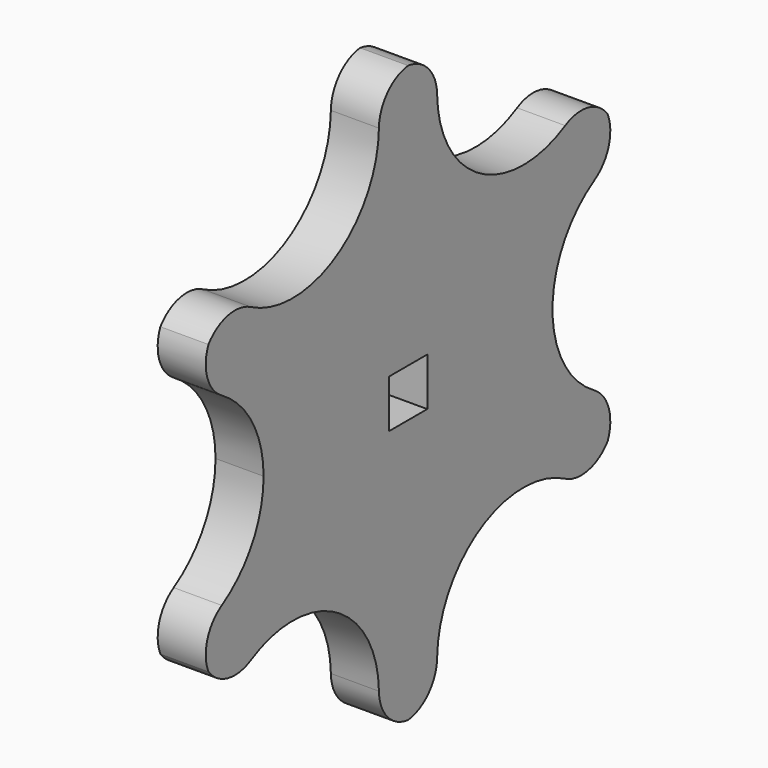
from build123d import *

# Parameters (mm, degrees)
F1_DEPTH    = 3.175
F2_W        = 3.175
F2_H        = 3.175
F3_DEPTH    = 25.4
F4_T1_DEPTH = 19.0841031127


# Not quite as in the source:
# - a fillet or chamfer that OpenCascade refuses, or shapes differently, is made with other operations: its cross-section is extruded or revolved along the edge and cut away or added


with BuildPart() as f1:
    # F0 (on Right) → F1 (new body)
    with BuildSketch(Plane.YZ):
        with BuildLine():
            ThreePointArc((17.7183197491, -6.9974027515), (11.9270078227, 0), (17.7183197491, 6.9974027515))
            ThreePointArc((17.7183197491, 6.9974027515), (16.4977839421, 9.525), (14.9190884179, 11.8458136394))
            ThreePointArc((14.9190884179, 11.8458136394), (5.9635039114, 10.3290917656), (2.7992313312, 18.8432163909))
            ThreePointArc((2.7992313312, 18.8432163909), (0, 19.05), (-2.7992313312, 18.8432163909))
            ThreePointArc((-2.7992313312, 18.8432163909), (-2.5020157635, 17.6871997533), (-2.4020078227, 16.4977839421))
            ThreePointArc((-2.4020078227, 16.4977839421), (-7.0435721899, 9.8209932773), (-14.9190884179, 11.8458136394))
            ThreePointArc((-14.9190884179, 11.8458136394), (-16.4977839421, 9.525), (-17.7183197491, 6.9974027515))
            ThreePointArc((-17.7183197491, 6.9974027515), (-13.5626251464, 4.5415564264), (-11.9270078227, 0))
            ThreePointArc((-11.9270078227, 0), (-13.5626251464, -4.5415564264), (-17.7183197491, -6.9974027515))
            ThreePointArc((-17.7183197491, -6.9974027515), (-16.4977839421, -9.525), (-14.9190884179, -11.8458136394))
            ThreePointArc((-14.9190884179, -11.8458136394), (-7.0435721899, -9.8209932773), (-2.4020078227, -16.4977839421))
            ThreePointArc((-2.4020078227, -16.4977839421), (-2.5020157635, -17.6871997533), (-2.7992313312, -18.8432163909))
            ThreePointArc((-2.7992313312, -18.8432163909), (0, -19.05), (2.7992313312, -18.8432163909))
            ThreePointArc((2.7992313312, -18.8432163909), (5.9635039114, -10.3290917656), (14.9190884179, -11.8458136394))
            ThreePointArc((14.9190884179, -11.8458136394), (16.4977839421, -9.525), (17.7183197491, -6.9974027515))
        make_face()
    extrude(amount=F1_DEPTH)

    # F2 (on face) → F3 (cut)
    with BuildSketch(Plane(origin=(0, 0, 0), x_dir=(0, -1, 0), z_dir=(-1, 0, 0))):
        Rectangle(F2_W, F2_H)
    extrude(amount=-F3_DEPTH, mode=Mode.SUBTRACT)

    # F4: fillet of radius 2.7258813335 on 12 edges, made by hand

    # F4_s2 → F4_t1 (cut)
    with BuildSketch(Plane.YZ.offset(-7.9545515563)):
        with BuildLine():
            ThreePointArc((-16.6826195947, 9.1974291766), (-15.0505041811, 10.5005937812), (-12.9751564545, 10.2661358457))
            ThreePointArc((-12.9751564545, 10.2661358457), (-14.0171055557, 10.9698543809), (-14.9190884179, 11.8458136394))
            ThreePointArc((-14.9190884179, 11.8458136394), (-15.8562439561, 10.5585049892), (-16.6826195947, 9.1974291766))
        make_face()
        with BuildLine():
            ThreePointArc((-15.3783126684, 6.1037471848), (-16.6190330599, 7.78382207), (-16.3065171138, 9.8488577824))
            ThreePointArc((-16.3065171138, 9.8488577824), (-17.0720555246, 8.45265758), (-17.7183197491, 6.9974027515))
            ThreePointArc((-17.7183197491, 6.9974027515), (-16.5087253475, 6.6542423084), (-15.3783126684, 6.1037471848))
        make_face()
        with BuildLine():
            ThreePointArc((-16.3065171138, -9.8488577824), (-16.6190330599, -7.78382207), (-15.3783126684, -6.1037471848))
            ThreePointArc((-15.3783126684, -6.1037471848), (-16.5087253475, -6.6542423084), (-17.7183197491, -6.9974027515))
            ThreePointArc((-17.7183197491, -6.9974027515), (-17.0720555246, -8.45265758), (-16.3065171138, -9.8488577824))
        make_face()
        with BuildLine():
            ThreePointArc((-12.9751564545, -10.2661358457), (-15.0505041811, -10.5005937812), (-16.6826195947, -9.1974291766))
            ThreePointArc((-16.6826195947, -9.1974291766), (-15.8562439561, -10.5585049892), (-14.9190884179, -11.8458136394))
            ThreePointArc((-14.9190884179, -11.8458136394), (-14.0171055557, -10.9698543809), (-12.9751564545, -10.2661358457))
        make_face()
        with BuildLine():
            ThreePointArc((-2.4031562138, -16.3698830306), (-1.5685288788, -18.2844158512), (0.3761024809, -19.046286959))
            ThreePointArc((0.3761024809, -19.046286959), (-1.2158115686, -19.0111625691), (-2.7992313312, -18.8432163909))
            ThreePointArc((-2.7992313312, -18.8432163909), (-2.4916197918, -17.6240966892), (-2.4031562138, -16.3698830306))
        make_face()
        with BuildLine():
            ThreePointArc((-2.4031562138, 16.3698830306), (-1.5685288788, 18.2844158512), (0.3761024809, 19.046286959))
            ThreePointArc((0.3761024809, 19.046286959), (-1.2158115686, 19.0111625691), (-2.7992313312, 18.8432163909))
            ThreePointArc((-2.7992313312, 18.8432163909), (-2.4916197918, 17.6240966892), (-2.4031562138, 16.3698830306))
        make_face()
        with BuildLine():
            ThreePointArc((16.6826195947, 9.1974291766), (15.0505041811, 10.5005937812), (12.9751564545, 10.2661358457))
            ThreePointArc((12.9751564545, 10.2661358457), (14.0171055557, 10.9698543809), (14.9190884179, 11.8458136394))
            ThreePointArc((14.9190884179, 11.8458136394), (15.8562439561, 10.5585049892), (16.6826195947, 9.1974291766))
        make_face()
        with BuildLine():
            ThreePointArc((-0.3761024809, 19.046286959), (1.5685288788, 18.2844158512), (2.4031562138, 16.3698830306))
            ThreePointArc((2.4031562138, 16.3698830306), (2.4916197918, 17.6240966892), (2.7992313312, 18.8432163909))
            ThreePointArc((2.7992313312, 18.8432163909), (1.2158115686, 19.0111625691), (-0.3761024809, 19.046286959))
        make_face()
        with BuildLine():
            ThreePointArc((15.3783126684, 6.1037471848), (16.6190330599, 7.78382207), (16.3065171138, 9.8488577824))
            ThreePointArc((16.3065171138, 9.8488577824), (17.0720555246, 8.45265758), (17.7183197491, 6.9974027515))
            ThreePointArc((17.7183197491, 6.9974027515), (16.5087253475, 6.6542423084), (15.3783126684, 6.1037471848))
        make_face()
        with BuildLine():
            ThreePointArc((16.3065171138, -9.8488577824), (16.6190330599, -7.78382207), (15.3783126684, -6.1037471848))
            ThreePointArc((15.3783126684, -6.1037471848), (16.5087253475, -6.6542423084), (17.7183197491, -6.9974027515))
            ThreePointArc((17.7183197491, -6.9974027515), (17.0720555246, -8.45265758), (16.3065171138, -9.8488577824))
        make_face()
        with BuildLine():
            ThreePointArc((12.9751564545, -10.2661358457), (15.0505041811, -10.5005937812), (16.6826195947, -9.1974291766))
            ThreePointArc((16.6826195947, -9.1974291766), (15.8562439561, -10.5585049892), (14.9190884179, -11.8458136394))
            ThreePointArc((14.9190884179, -11.8458136394), (14.0171055557, -10.9698543809), (12.9751564545, -10.2661358457))
        make_face()
        with BuildLine():
            ThreePointArc((-0.3761024809, -19.046286959), (1.5685288788, -18.2844158512), (2.4031562138, -16.3698830306))
            ThreePointArc((2.4031562138, -16.3698830306), (2.4916197918, -17.6240966892), (2.7992313312, -18.8432163909))
            ThreePointArc((2.7992313312, -18.8432163909), (1.2158115686, -19.0111625691), (-0.3761024809, -19.046286959))
        make_face()
    extrude(amount=F4_T1_DEPTH, mode=Mode.SUBTRACT)


solid = f1.part
